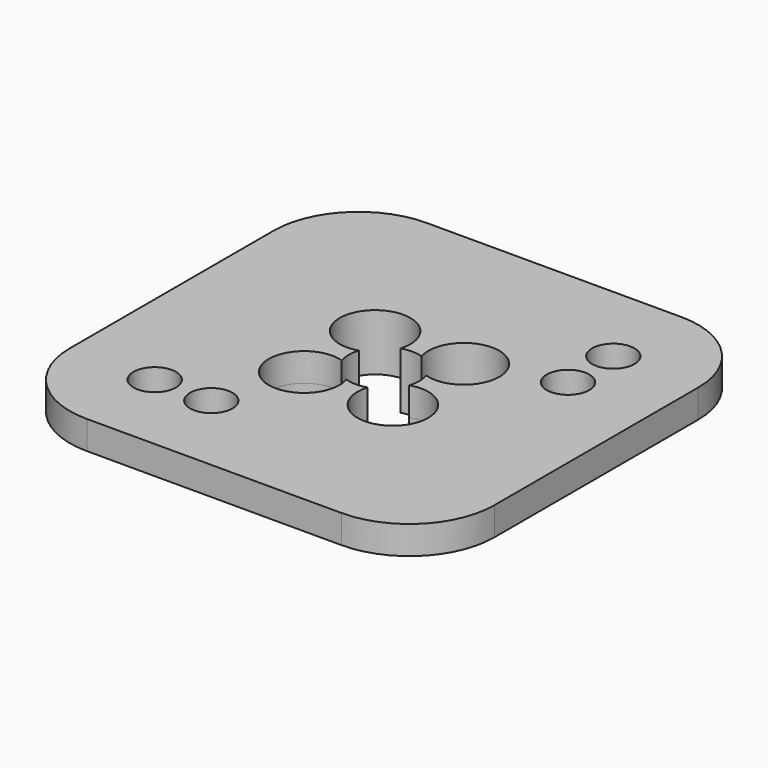
from build123d import *
from build123d import SkipClean  # not in build123d's __all__

# Parameters (mm, degrees)
F0_R     = 4
F1_DEPTH = 1
F2_W     = 15
F2_H     = 15
F2_R     = 5
F2_R_2   = 4
F3_DEPTH = 1
F4_R     = 3
F5_R     = 0.75
F6_DEPTH = 25


# Not quite as in the source:
# - after a boolean that leaves OpenCascade's solid faulty, fix() repairs it


with BuildPart() as f1:
    # F0 (on Top) → F1 (new body)
    with BuildSketch(Plane.XY):
        Circle(F0_R)
        with BuildLine():
            ThreePointArc((1.1922665017, 0.3755004513), (1.2354823202, 0.1899564067), (1.25, 0))
            ThreePointArc((1.25, 0), (1.2354823202, -0.1899564067), (1.1922665017, -0.3755004513))
            ThreePointArc((1.1922665017, -0.3755004513), (2.3070654164, -0.559829563), (2.817766953, -1.567766953))
            ThreePointArc((2.817766953, -1.567766953), (1.3778105463, -2.8032492732), (0.3755004513, -1.1922665017))
            ThreePointArc((0.3755004513, -1.1922665017), (0, -1.25), (-0.3755004513, -1.1922665017))
            ThreePointArc((-0.3755004513, -1.1922665017), (-0.3322846327, -1.3778105463), (-0.317766953, -1.567766953))
            ThreePointArc((-0.317766953, -1.567766953), (-2.5757043429, -2.3070654164), (-1.1922665017, -0.3755004513))
            ThreePointArc((-1.1922665017, -0.3755004513), (-1.25, 0), (-1.1922665017, 0.3755004513))
            ThreePointArc((-1.1922665017, 0.3755004513), (-2.5757043429, 2.3070654164), (-0.317766953, 1.567766953))
            ThreePointArc((-0.317766953, 1.567766953), (-0.3322846327, 1.3778105463), (-0.3755004513, 1.1922665017))
            ThreePointArc((-0.3755004513, 1.1922665017), (0, 1.25), (0.3755004513, 1.1922665017))
            ThreePointArc((0.3755004513, 1.1922665017), (1.3778105463, 2.8032492732), (2.817766953, 1.567766953))
            ThreePointArc((2.817766953, 1.567766953), (2.3070654164, 0.559829563), (1.1922665017, 0.3755004513))
        make_face(mode=Mode.SUBTRACT)
    extrude(amount=-F1_DEPTH)

    # F2 (on face) → F3 (join)
    with BuildSketch(Plane.XY):
        Rectangle(F2_W, F2_H)
        Circle(F2_R, mode=Mode.SUBTRACT)
        Circle(F2_R)
        Circle(F2_R_2, mode=Mode.SUBTRACT)
        Circle(F2_R_2)
        with BuildLine():
            ThreePointArc((1.1922665017, 0.3755004513), (1.2354823202, 0.1899564067), (1.25, 0))
            ThreePointArc((1.25, 0), (1.2354823202, -0.1899564067), (1.1922665017, -0.3755004513))
            ThreePointArc((1.1922665017, -0.3755004513), (2.4516504294, -2.4516504294), (0.3755004513, -1.1922665017))
            ThreePointArc((0.3755004513, -1.1922665017), (0, -1.25), (-0.3755004513, -1.1922665017))
            ThreePointArc((-0.3755004513, -1.1922665017), (-2.4516504294, -2.4516504294), (-1.1922665017, -0.3755004513))
            ThreePointArc((-1.1922665017, -0.3755004513), (-1.25, 0), (-1.1922665017, 0.3755004513))
            ThreePointArc((-1.1922665017, 0.3755004513), (-2.5757043429, 2.3070654164), (-0.317766953, 1.567766953))
            ThreePointArc((-0.317766953, 1.567766953), (-0.3322846327, 1.3778105463), (-0.3755004513, 1.1922665017))
            ThreePointArc((-0.3755004513, 1.1922665017), (0, 1.25), (0.3755004513, 1.1922665017))
            ThreePointArc((0.3755004513, 1.1922665017), (1.3778105463, 2.8032492732), (2.817766953, 1.567766953))
            ThreePointArc((2.817766953, 1.567766953), (2.3070654164, 0.559829563), (1.1922665017, 0.3755004513))
        make_face(mode=Mode.SUBTRACT)
    with SkipClean():  # cleaning this boolean's faces spoils the solid; the shape is the same uncleaned
        extrude(amount=F3_DEPTH)

    # F4
    f4_edges = [f1.edges().sort_by_distance(p)[0] for p in [
        (-7.5, -7.5, 0.5),
        (7.5, -7.5, 0.5),
        (-7.5, 7.5, 0.5),
        (7.5, 7.5, 0.5),
    ]]
    fillet(f4_edges, radius=F4_R)

    # F5 (on face) → F6 (cut)
    with BuildSketch(Plane(origin=(0, 0, 0), x_dir=(1, 0, 0), z_dir=(0, 0, -1))):
        with Locations((-4.5, 4.5)):
            Circle(F5_R)
        with Locations((-2.5, 4.5)):
            Circle(F5_R)
        with Locations((4.5, -4.5)):
            Circle(F5_R)
        with Locations((4.5, -2.5)):
            Circle(F5_R)
    extrude(amount=-F6_DEPTH, mode=Mode.SUBTRACT)

    add(f1.part.fix(), mode=Mode.REPLACE)


solid = f1.part
